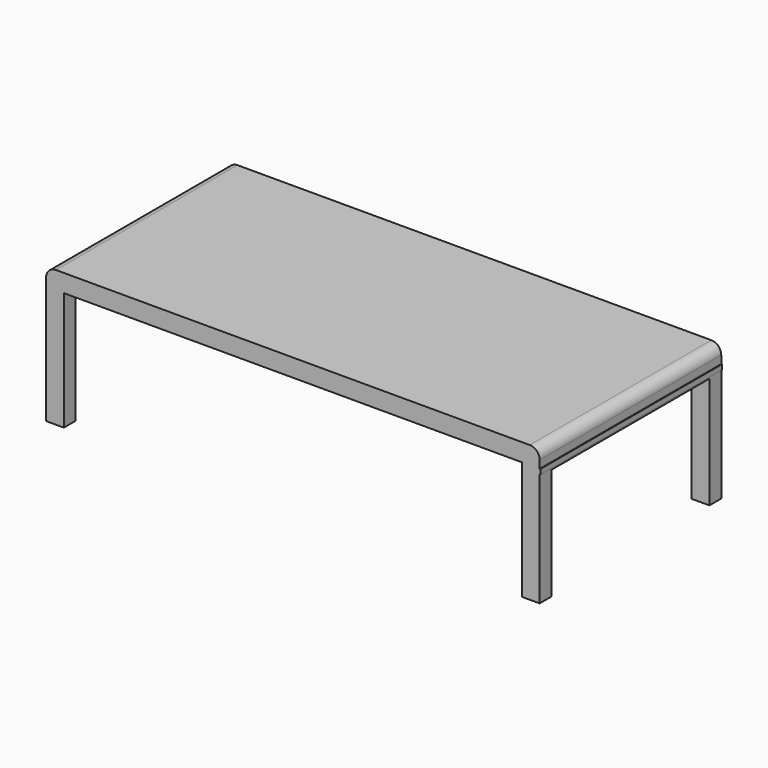
from build123d import *

# Parameters (mm, degrees)
F0_W     = 18
F0_H     = 120
F1_DEPTH = 115
F2_R     = 10
F3_W     = 200
F3_H     = 113
F4_DEPTH = 500.001
F5_W     = 18.0844597816
F5_H     = 229.7550716996
F5_W_2   = 18.6774961948
F5_H_2   = 230
F6_DEPTH = 5


with BuildPart() as f1:
    # F0 (on Front) → F1 (new body, symmetric)
    with BuildSketch(Plane.XZ):
        Polygon((250, 9), (-250, 9), (-250, -9), (-232, -9), (232, -9), (250, -9), align=None)
        with Locations((-241, -69)):
            Rectangle(F0_W, F0_H)
        with Locations((241, -69)):
            Rectangle(F0_W, F0_H)
    extrude(amount=F1_DEPTH, both=True)

    # F2
    f2_edges = [f1.edges().sort_by_distance(p)[0] for p in [
        (-250, 0, 9),
        (250, 0, 9),
    ]]
    fillet(f2_edges, radius=F2_R)

    # F3 (on face) → F4 (cut, through all)
    with BuildSketch(Plane.YZ.offset(250)):
        with Locations((0, -72.5)):
            Rectangle(F3_W, F3_H)
    extrude(amount=-F4_DEPTH, mode=Mode.SUBTRACT)

    # F5 (on face) → F6 (join)
    with BuildSketch(Plane(origin=(0, 0, -9), x_dir=(1, 0, 0), z_dir=(0, 0, -1))):
        with Locations((-241.0422298908, -0.1224641502)):
            Rectangle(F5_W, F5_H)
        with Locations((241.3387480974, 0)):
            Rectangle(F5_W_2, F5_H_2)
    extrude(amount=F6_DEPTH)


solid = f1.part
